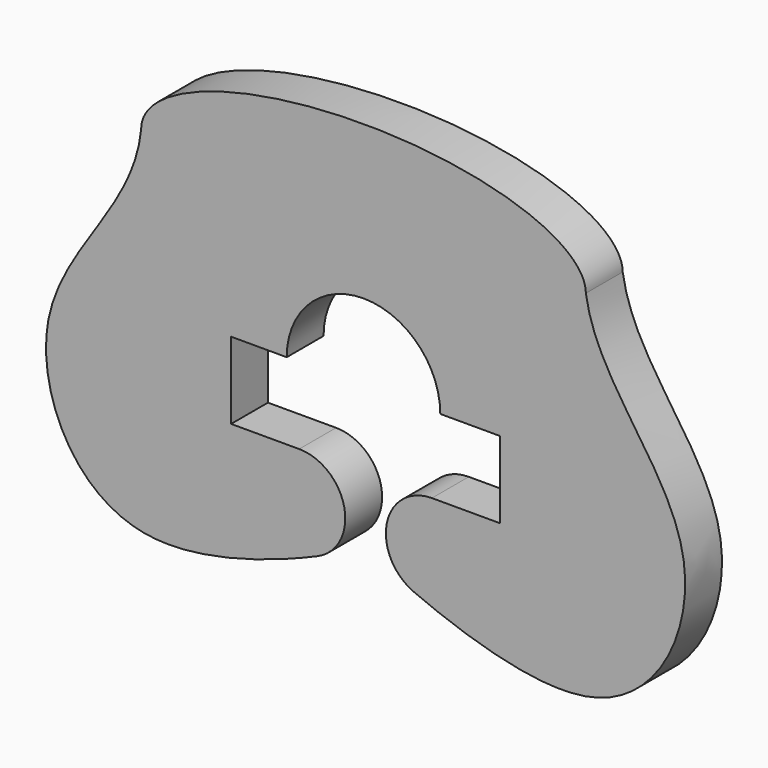
from build123d import *

# Parameters (mm, degrees)
F1_DEPTH = 3


# Not quite as in the source:
# - ends of sketch curves that miss each other by under 0.0002 mm in the source are joined
# - the dataset's text gives a spline's control points without its knots; the knots are read off the source's solid


with BuildPart() as f1:
    # F0 (on Front) → F1 (new body)
    with BuildSketch(Plane.XZ):
        with BuildLine():
            Line((-4.321138, -5.882648), (-8.755, -5.882648))
            Line((-8.755, -5.882648), (-8.755, -0.882648))
            Line((-8.755, -0.882648), (-5.134039, -0.882648))
            ThreePointArc((-5.134039, -0.882648), (-0.134039, 4.117352), (4.865961, -0.882648))
            Line((4.865961, -0.882648), (8.755, -0.882648))
            Line((8.755, -0.882648), (8.755, -5.882648))
            Line((8.755, -5.882648), (4.321137, -5.882648))
            ThreePointArc((4.321137, -5.882648), (1.3830953266, -8.2760912214), (3.1330776048, -11.6373739162))
            add(Edge.make_bspline(
                [(14.341757, 9.117352), (15.09434, 4.111526), (24.07864, -2.094143), (17.273633, -16.953755), (5.88345, -12.823555), (3.1330776048, -11.6373739162)],
                knots=[28.987347, 28.987347, 28.987347, 28.987347, 42.872008, 54.1154, 62.665306, 62.665306, 62.665306, 62.665306], degree=3))
            add(Edge.make_bspline(
                [(14.341757, 9.117352), (14.341757, 14.117352866), (-0.1340415073, 14.117352), (-14.6098400146, 14.117351134), (-14.609835, 9.1173502679)],
                knots=[0, 0, 0, 1.5707965, 1.5707965, 3.141593, 3.141593, 3.141593], degree=2, weights=[1, 0.7071067199, 1, 0.7071067199, 1]))
            add(Edge.make_bspline(
                [(-14.609835, 9.1173502679), (-15.094341, 4.111526), (-24.078641, -2.094143), (-17.273634, -16.953755), (-5.883451, -12.823555), (-3.133078, -11.637373)],
                knots=[28.987347, 28.987347, 28.987347, 28.987347, 42.872008, 54.1154, 62.665306, 62.665306, 62.665306, 62.665306], degree=3))
            ThreePointArc((-3.133078, -11.637373), (-1.3830964195, -8.2760907718), (-4.321138, -5.882648))
        make_face()
    extrude(amount=F1_DEPTH)


solid = f1.part
